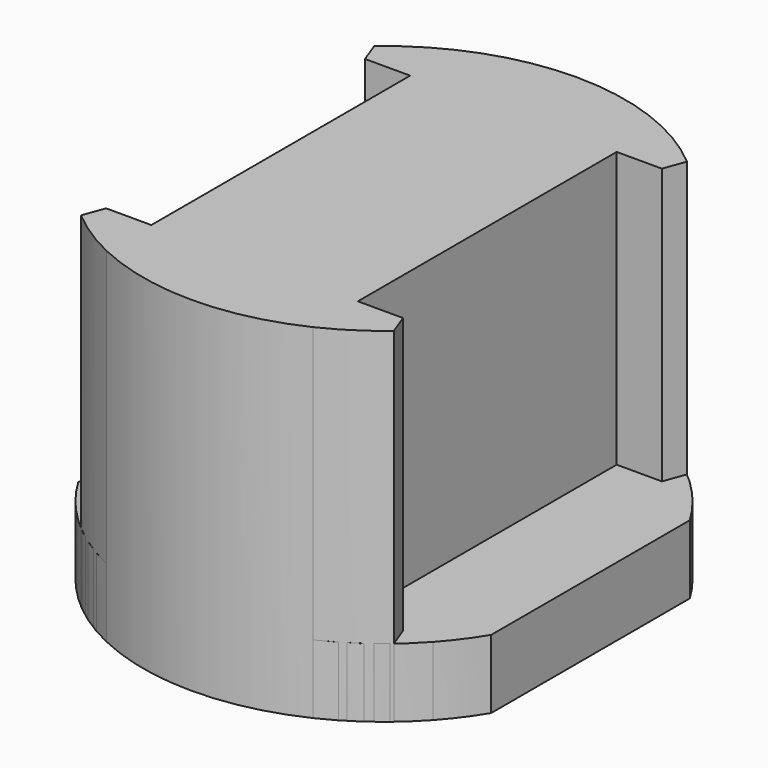
from build123d import *

# Parameters (mm, degrees)
F1_DEPTH    = 5
F0_W        = 6.6
F0_H        = 1.5
F0_W_2      = 4.2
F0_H_2      = 23.5
F2_DEPTH    = 25
F3_DEPTH    = 15.6
F4_T1_DEPTH = 36.3750267574


# Not quite as in the source:
# - a fillet or chamfer that OpenCascade refuses, or shapes differently, is made with other operations: its cross-section is extruded or revolved along the edge and cut away or added


with BuildPart() as f1:
    # F0 (on Top) → F1 (new body)
    with BuildSketch(Plane.XY):
        with BuildLine():
            Line((15, -9.0138781887), (15, 9.0138781887))
            ThreePointArc((15, 9.0138781887), (14.0511141288, 10.4314999755), (12.9687123493, 11.75))
            Line((12.9687123493, 11.75), (7.5, 11.75))
            Line((7.5, 11.75), (7.5, -11.75))
            Line((7.5, -11.75), (12.9687123493, -11.75))
            ThreePointArc((12.9687123493, -11.75), (14.0511141288, -10.4314999755), (15, -9.0138781887))
        make_face()
        with BuildLine():
            ThreePointArc((7.5, -15.8113883008), (10.4338758399, -14.0493499834), (12.9687123493, -11.75))
            Line((12.9687123493, -11.75), (7.5, -11.75))
            Line((7.5, -11.75), (7.5, -15.8113883008))
        make_face()
        with BuildLine():
            Line((7.5, 11.75), (12.9687123493, 11.75))
            ThreePointArc((12.9687123493, 11.75), (10.4338758399, 14.0493499834), (7.5, 15.8113883008))
            Line((7.5, 15.8113883008), (7.5, 11.75))
        make_face()
    extrude(amount=F1_DEPTH)


with BuildPart() as f1b:
    # F0 (on Top) → F1, piece 2 (new body)
    with BuildSketch(Plane.XY):
        with BuildLine():
            Line((-7.5, 11.75), (-12.9687123493, 11.75))
            ThreePointArc((-12.9687123493, 11.75), (-14.0511141288, 10.4314999755), (-15, 9.0138781887))
            Line((-15, 9.0138781887), (-15, -9.0138781887))
            ThreePointArc((-15, -9.0138781887), (-14.0511141288, -10.4314999755), (-12.9687123493, -11.75))
            Line((-12.9687123493, -11.75), (-7.5, -11.75))
            Line((-7.5, -11.75), (-7.5, 11.75))
        make_face()
        with BuildLine():
            Line((-7.5, 11.75), (-7.5, 15.8113883008))
            ThreePointArc((-7.5, 15.8113883008), (-10.4338758399, 14.0493499834), (-12.9687123493, 11.75))
            Line((-12.9687123493, 11.75), (-7.5, 11.75))
        make_face()
        with BuildLine():
            ThreePointArc((-12.9687123493, -11.75), (-10.4338758399, -14.0493499834), (-7.5, -15.8113883008))
            Line((-7.5, -15.8113883008), (-7.5, -11.75))
            Line((-7.5, -11.75), (-12.9687123493, -11.75))
        make_face()
    extrude(amount=F1_DEPTH)


with BuildPart() as f2:
    # F0 (on Top) → F2 (new body)
    with BuildSketch(Plane.XY):
        with Locations((0, 12.5)):
            Rectangle(F0_W, F0_H)
        with BuildLine():
            Line((7.5, 11.75), (7.5, 15.8113883008))
            ThreePointArc((7.5, 15.8113883008), (0, 17.5), (-7.5, 15.8113883008))
            Line((-7.5, 15.8113883008), (-7.5, 11.75))
            Line((-7.5, 11.75), (-3.3, 11.75))
            Line((-3.3, 11.75), (-3.3, 13.25))
            Line((-3.3, 13.25), (3.3, 13.25))
            Line((3.3, 13.25), (3.3, 11.75))
            Line((3.3, 11.75), (7.5, 11.75))
        make_face()
        with Locations((-5.4, 0)):
            Rectangle(F0_W_2, F0_H_2)
        with BuildLine():
            ThreePointArc((-7.5, -15.8113883008), (0, -17.5), (7.5, -15.8113883008))
            Line((7.5, -15.8113883008), (7.5, -11.75))
            Line((7.5, -11.75), (3.3, -11.75))
            Line((3.3, -11.75), (3.3, -13.25))
            Line((3.3, -13.25), (-3.3, -13.25))
            Line((-3.3, -13.25), (-3.3, -11.75))
            Line((-3.3, -11.75), (-7.5, -11.75))
            Line((-7.5, -11.75), (-7.5, -15.8113883008))
        make_face()
        with Locations((5.4, 0)):
            Rectangle(F0_W_2, F0_H_2)
        Rectangle(F0_W, F0_H_2)
        with Locations((0, -12.5)):
            Rectangle(F0_W, F0_H)
        with BuildLine():
            ThreePointArc((-12.9687123493, -11.75), (-10.4338758399, -14.0493499834), (-7.5, -15.8113883008))
            Line((-7.5, -15.8113883008), (-7.5, -11.75))
            Line((-7.5, -11.75), (-12.9687123493, -11.75))
        make_face()
        with BuildLine():
            Line((-7.5, 11.75), (-7.5, 15.8113883008))
            ThreePointArc((-7.5, 15.8113883008), (-10.4338758399, 14.0493499834), (-12.9687123493, 11.75))
            Line((-12.9687123493, 11.75), (-7.5, 11.75))
        make_face()
        with BuildLine():
            Line((7.5, 11.75), (12.9687123493, 11.75))
            ThreePointArc((12.9687123493, 11.75), (10.4338758399, 14.0493499834), (7.5, 15.8113883008))
            Line((7.5, 15.8113883008), (7.5, 11.75))
        make_face()
        with BuildLine():
            ThreePointArc((7.5, -15.8113883008), (10.4338758399, -14.0493499834), (12.9687123493, -11.75))
            Line((12.9687123493, -11.75), (7.5, -11.75))
            Line((7.5, -11.75), (7.5, -15.8113883008))
        make_face()
    extrude(amount=F2_DEPTH)

    # F0 (on Top) → F3 (cut)
    with BuildSketch(Plane.XY):
        with Locations((0, 12.5)):
            Rectangle(F0_W, F0_H)
        Rectangle(F0_W, F0_H_2)
        with Locations((0, -12.5)):
            Rectangle(F0_W, F0_H)
    extrude(amount=F3_DEPTH, mode=Mode.SUBTRACT)

    # F4: chamfer of 2 on 4 edges, made by hand

    # F4_s2 → F4_t1 (cut)
    with BuildSketch(Plane.XY.offset(-5.6875133787)):
        with BuildLine():
            Line((-10.7571586121, -11.6749396443), (-11.3881617362, -13.3863096005))
            Line((-11.3881617362, -13.3863096005), (-11.4141285615, -13.4167353131))
            ThreePointArc((-11.4141285615, -13.4167353131), (-12.2058182488, -12.5964122224), (-12.9983551204, -11.7768571429))
            Line((-12.9983551204, -11.7768571429), (-12.9687123493, -11.71))
            ThreePointArc((-12.9687123493, -11.71), (-11.8629354807, -11.71), (-10.7571586121, -11.6349396443))
            Line((-10.7571586121, -11.6349396443), (-10.7571586121, -11.6749396443))
        make_face()
        with BuildLine():
            Line((11.3881617362, -13.3863096005), (10.7571586121, -11.6749396443))
            Line((10.7571586121, -11.6749396443), (10.7571586121, -11.6349396443))
            ThreePointArc((10.7571586121, -11.6349396443), (11.8629354807, -11.71), (12.9687123493, -11.71))
            Line((12.9687123493, -11.71), (12.9983551204, -11.7768571429))
            ThreePointArc((12.9983551204, -11.7768571429), (12.2058182488, -12.5964122224), (11.4141285615, -13.4167353131))
            Line((11.4141285615, -13.4167353131), (11.3881617362, -13.3863096005))
        make_face()
        with BuildLine():
            Line((11.3881617362, 13.3863096005), (10.7571586121, 11.6749396443))
            Line((10.7571586121, 11.6749396443), (10.7571586121, 11.6349396443))
            ThreePointArc((10.7571586121, 11.6349396443), (11.8629354807, 11.71), (12.9687123493, 11.71))
            Line((12.9687123493, 11.71), (12.9983551204, 11.7768571429))
            ThreePointArc((12.9983551204, 11.7768571429), (12.2058182488, 12.5964122224), (11.4141285615, 13.4167353131))
            Line((11.4141285615, 13.4167353131), (11.3881617362, 13.3863096005))
        make_face()
        with BuildLine():
            Line((-10.7571586121, 11.6749396443), (-11.3881617362, 13.3863096005))
            Line((-11.3881617362, 13.3863096005), (-11.4141285615, 13.4167353131))
            ThreePointArc((-11.4141285615, 13.4167353131), (-12.2058182488, 12.5964122224), (-12.9983551204, 11.7768571429))
            Line((-12.9983551204, 11.7768571429), (-12.9687123493, 11.71))
            ThreePointArc((-12.9687123493, 11.71), (-11.8629354807, 11.71), (-10.7571586121, 11.6349396443))
            Line((-10.7571586121, 11.6349396443), (-10.7571586121, 11.6749396443))
        make_face()
    extrude(amount=F4_T1_DEPTH, mode=Mode.SUBTRACT)


solid = Compound([f1.part, f1b.part, f2.part])
